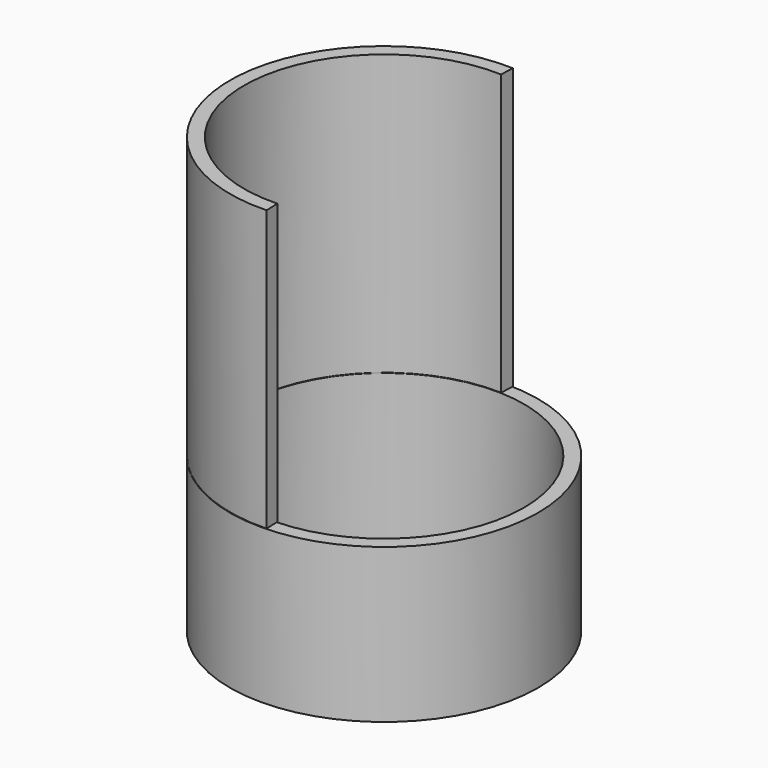
from build123d import *

# Parameters (mm, degrees)
F0_R          = 27.5
F0_R_2        = 25
F1_DEPTH      = 27.5
F2_W          = 2.5
F2_H          = 50
F3_ANGLE_BACK = 92.1160547881
F3_ANGLE      = 184.2321095762


# Not quite as in the source:
# - a feature of the source that left no trace in its solid (it failed there, or was rolled back) is left out


with BuildPart() as f1:
    # F0 (on Top) → F1 (new body)
    with BuildSketch(Plane.XY):
        Circle(F0_R)
        Circle(F0_R_2, mode=Mode.SUBTRACT)
    extrude(amount=F1_DEPTH)


with BuildPart() as f3:
    # F2 (on Front) → F3 (revolve)
    with BuildSketch(Plane.XZ, mode=Mode.PRIVATE) as f3_sk:
        with Locations((-26.2295312434, 52.5726281106)):
            Rectangle(F2_W, F2_H)
    revolve(f3_sk.sketch.rotate(Axis((0, 0, 0), (0, 0, -1)), -F3_ANGLE_BACK), axis=Axis((0, 0, 0), (0, 0, -1)), revolution_arc=F3_ANGLE)


solid = Compound([f1.part, f3.part])
